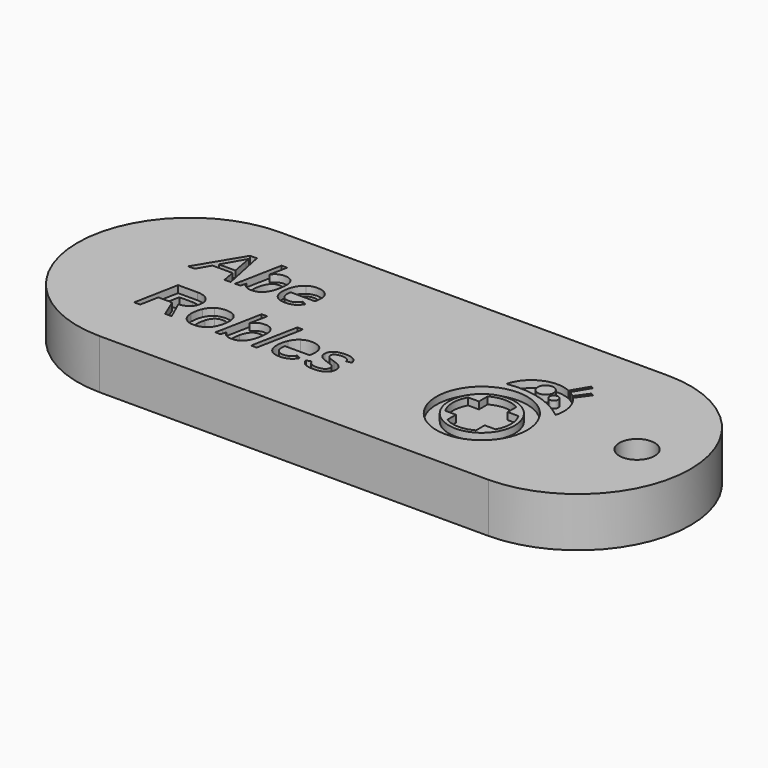
from build123d import *

# Parameters (mm, degrees)
F0_R         = 8.1541463089
F0_R_2       = 3.175
F1_DEPTH     = 8.89
F0_TEXT_SIZE = 11.5409836066
F2_DEPTH     = 7.62
F0_R_3       = 5.9091517201
F0_R_4       = 0.7843933306
F0_R_5       = 1.4228643603
F3_DEPTH     = 7.62
F4_DEPTH     = 8.89


# Not quite as in the source:
# - Text() gives the source's letters only with a copy of the font that has no kerning and outlines rounded to 1/6400 em; it was checked with that copy


with BuildPart() as f1:
    # F0 (on Top) → F1 (new body)
    with BuildSketch(Plane.XY):
        with BuildLine():
            ThreePointArc((34.925, -20.2309455037), (55.0719912037, 0), (34.925, 20.2309455037))
            Line((34.925, 20.2309455037), (34.7567415551, 20.2309455037))
            Line((34.7567415551, 20.2309455037), (-34.7567415551, 20.2309455037))
            Line((-34.7567415551, 20.2309455037), (-34.925, 20.2309455037))
            ThreePointArc((-34.925, 20.2309455037), (-55.0719912037, 0), (-34.925, -20.2309455037))
            Line((-34.925, -20.2309455037), (-34.7567415551, -20.2309455037))
            Line((-34.7567415551, -20.2309455037), (34.7567415551, -20.2309455037))
            Line((34.7567415551, -20.2309455037), (34.925, -20.2309455037))
        make_face()
        with BuildLine():
            Line((-30.8085259014, -9.1939333774), (-31.9698373768, -9.1939333774))
            Line((-31.9698373768, -9.1939333774), (-33.3385259014, -5.8975399348))
            Line((-33.3385259014, -5.8975399348), (-35.8234439342, -5.8975399348))
            Line((-35.8234439342, -5.8975399348), (-36.4600013112, -9.1939333774))
            Line((-36.4600013112, -9.1939333774), (-37.5365586883, -9.1939333774))
            Line((-37.5365586883, -9.1939333774), (-35.9983619669, -1.2540973119))
            Line((-35.9983619669, -1.2540973119), (-32.5486898358, -1.2540973119))
            add(Edge.make_bspline(
                [(-32.5486898358, -1.2540973119), (-31.3440996719, -1.2540973119), (-30.6281980325, -1.8284415742)],
                knots=[0, 0, 0, 1, 1, 1], degree=2))
            add(Edge.make_bspline(
                [(-30.6281980325, -1.8284415742), (-29.9122963932, -2.4027858364), (-29.9122963932, -3.3386874758)],
                knots=[0, 0, 0, 1, 1, 1], degree=2))
            add(Edge.make_bspline(
                [(-29.9122963932, -3.3386874758), (-29.9122963932, -4.3990153446), (-30.5209029505, -5.0184415742)],
                knots=[0, 0, 0, 1, 1, 1], degree=2))
            add(Edge.make_bspline(
                [(-30.5209029505, -5.0184415742), (-31.1295095079, -5.6378678037), (-32.3178701637, -5.8019661643)],
                knots=[0, 0, 0, 1, 1, 1], degree=2))
            Line((-32.3178701637, -5.8019661643), (-30.8085259014, -9.1939333774))
        make_face(mode=Mode.SUBTRACT)
        with BuildLine():
            add(Edge.make_bspline(
                [(-24.1300832784, -3.606474361), (-23.5052472128, -4.2240973119), (-23.5052472128, -5.3457366561)],
                knots=[0, 0, 0, 1, 1, 1], degree=2))
            add(Edge.make_bspline(
                [(-23.5052472128, -5.3457366561), (-23.5052472128, -6.0778678037), (-23.7306570489, -6.8695071479)],
                knots=[0, 0, 0, 1, 1, 1], degree=2))
            add(Edge.make_bspline(
                [(-23.7306570489, -6.8695071479), (-23.956066885, -7.6611464922), (-24.3753291801, -8.2102448528)],
                knots=[0, 0, 0, 1, 1, 1], degree=2))
            add(Edge.make_bspline(
                [(-24.3753291801, -8.2102448528), (-24.7945914751, -8.7593432135), (-25.4031980325, -9.0334415742)],
                knots=[0, 0, 0, 1, 1, 1], degree=2))
            add(Edge.make_bspline(
                [(-25.4031980325, -9.0334415742), (-26.0118045899, -9.3075399348), (-26.7908209833, -9.3075399348)],
                knots=[0, 0, 0, 1, 1, 1], degree=2))
            add(Edge.make_bspline(
                [(-26.7908209833, -9.3075399348), (-27.8944275407, -9.3075399348), (-28.5372963932, -8.6421300987)],
                knots=[0, 0, 0, 1, 1, 1], degree=2))
            add(Edge.make_bspline(
                [(-28.5372963932, -8.6421300987), (-29.1801652456, -7.9767202627), (-29.1801652456, -6.8334415742)],
                knots=[0, 0, 0, 1, 1, 1], degree=2))
            add(Edge.make_bspline(
                [(-29.1801652456, -6.8334415742), (-29.1567226227, -5.6829497709), (-28.7627062292, -4.7930317381)],
                knots=[0, 0, 0, 1, 1, 1], degree=2))
            add(Edge.make_bspline(
                [(-28.7627062292, -4.7930317381), (-28.3686898358, -3.9031137053), (-27.669919344, -3.4459825578)],
                knots=[0, 0, 0, 1, 1, 1], degree=2))
            add(Edge.make_bspline(
                [(-27.669919344, -3.4459825578), (-26.9711488522, -2.9888514102), (-25.9396734423, -2.9888514102)],
                knots=[0, 0, 0, 1, 1, 1], degree=2))
            add(Edge.make_bspline(
                [(-25.9396734423, -2.9888514102), (-24.754919344, -2.9888514102), (-24.1300832784, -3.606474361)],
                knots=[0, 0, 0, 1, 1, 1], degree=2))
        make_face(mode=Mode.SUBTRACT)
        with BuildLine():
            add(Edge.make_bspline(
                [(-20.0736078686, -3.2259825578), (-19.6173783604, -2.9834415742), (-18.9465586883, -2.9834415742)],
                knots=[0, 0, 0, 1, 1, 1], degree=2))
            add(Edge.make_bspline(
                [(-18.9465586883, -2.9834415742), (-18.0611488522, -2.9834415742), (-17.5679521309, -3.5163104266)],
                knots=[0, 0, 0, 1, 1, 1], degree=2))
            add(Edge.make_bspline(
                [(-17.5679521309, -3.5163104266), (-17.0747554096, -4.0491792791), (-17.0747554096, -4.9778678037)],
                knots=[0, 0, 0, 1, 1, 1], degree=2))
            add(Edge.make_bspline(
                [(-17.0747554096, -4.9778678037), (-17.0747554096, -6.1229497709), (-17.4218865571, -7.1959005905)],
                knots=[0, 0, 0, 1, 1, 1], degree=2))
            add(Edge.make_bspline(
                [(-17.4218865571, -7.1959005905), (-17.7690177046, -8.2688514102), (-18.3974603276, -8.7881956725)],
                knots=[0, 0, 0, 1, 1, 1], degree=2))
            add(Edge.make_bspline(
                [(-18.3974603276, -8.7881956725), (-19.0259029505, -9.3075399348), (-19.9996734423, -9.3075399348)],
                knots=[0, 0, 0, 1, 1, 1], degree=2))
            add(Edge.make_bspline(
                [(-19.9996734423, -9.3075399348), (-20.6939357374, -9.3075399348), (-21.127624262, -9.0136055086)],
                knots=[0, 0, 0, 1, 1, 1], degree=2))
            add(Edge.make_bspline(
                [(-21.127624262, -9.0136055086), (-21.5613127866, -8.7196710824), (-21.7416406555, -8.1913104266)],
                knots=[0, 0, 0, 1, 1, 1], degree=2))
            Line((-21.7416406555, -8.1913104266), (-21.7578701637, -8.1913104266))
            add(Edge.make_bspline(
                [(-21.7578701637, -8.1913104266), (-21.7975422948, -8.3986874758), (-21.8931160653, -8.7881956725)],
                knots=[0, 0, 0, 1, 1, 1], degree=2))
            add(Edge.make_bspline(
                [(-21.8931160653, -8.7881956725), (-21.9886898358, -9.1777038692), (-22.0013127866, -9.1939333774)],
                knots=[0, 0, 0, 1, 1, 1], degree=2))
            Line((-22.0013127866, -9.1939333774), (-22.9750832784, -9.1939333774))
            add(Edge.make_bspline(
                [(-22.9750832784, -9.1939333774), (-22.9480340981, -9.1091792791), (-22.8659849178, -8.7313923938)],
                knots=[0, 0, 0, 1, 1, 1], degree=2))
            add(Edge.make_bspline(
                [(-22.8659849178, -8.7313923938), (-22.7839357374, -8.3536055086), (-22.6991816391, -7.9370481315)],
                knots=[0, 0, 0, 1, 1, 1], degree=2))
            Line((-22.6991816391, -7.9370481315), (-21.3196734423, -0.8303268201))
            Line((-21.3196734423, -0.8303268201), (-20.3044275407, -0.8303268201))
            Line((-20.3044275407, -0.8303268201), (-20.771476721, -3.2142612463))
            add(Edge.make_bspline(
                [(-20.771476721, -3.2142612463), (-20.8165586883, -3.4739333774), (-20.9644275407, -4.0040973119)],
                knots=[0, 0, 0, 1, 1, 1], degree=2))
            Line((-20.9644275407, -4.0040973119), (-20.9409849178, -4.0040973119))
            add(Edge.make_bspline(
                [(-20.9409849178, -4.0040973119), (-20.5298373768, -3.4685235414), (-20.0736078686, -3.2259825578)],
                knots=[0, 0, 0, 1, 1, 1], degree=2))
        make_face(mode=Mode.SUBTRACT)
        with BuildLine():
            Line((-8.3018045899, -6.3591792791), (-12.7144275407, -6.3591792791))
            add(Edge.make_bspline(
                [(-12.7144275407, -6.3591792791), (-12.7486898358, -6.5557366561), (-12.764919344, -6.9957366561)],
                knots=[0, 0, 0, 1, 1, 1], degree=2))
            add(Edge.make_bspline(
                [(-12.764919344, -6.9957366561), (-12.764919344, -7.7459005905), (-12.3898373768, -8.1462284594)],
                knots=[0, 0, 0, 1, 1, 1], degree=2))
            add(Edge.make_bspline(
                [(-12.3898373768, -8.1462284594), (-12.0147554096, -8.5465563283), (-11.2609849178, -8.5465563283)],
                knots=[0, 0, 0, 1, 1, 1], degree=2))
            add(Edge.make_bspline(
                [(-11.2609849178, -8.5465563283), (-10.7145914751, -8.5465563283), (-10.2691816391, -8.276064525)],
                knots=[0, 0, 0, 1, 1, 1], degree=2))
            add(Edge.make_bspline(
                [(-10.2691816391, -8.276064525), (-9.823771803, -8.0055727217), (-9.574919344, -7.5367202627)],
                knots=[0, 0, 0, 1, 1, 1], degree=2))
            Line((-9.574919344, -7.5367202627), (-8.7977062292, -7.8919661643))
            add(Edge.make_bspline(
                [(-8.7977062292, -7.8919661643), (-9.2088537702, -8.6295071479), (-9.8427062292, -8.9685235414)],
                knots=[0, 0, 0, 1, 1, 1], degree=2))
            add(Edge.make_bspline(
                [(-9.8427062292, -8.9685235414), (-10.4765586883, -9.3075399348), (-11.3781980325, -9.3075399348)],
                knots=[0, 0, 0, 1, 1, 1], degree=2))
            add(Edge.make_bspline(
                [(-11.3781980325, -9.3075399348), (-12.5106570489, -9.3075399348), (-13.1390996719, -8.6790973119)],
                knots=[0, 0, 0, 1, 1, 1], degree=2))
            add(Edge.make_bspline(
                [(-13.1390996719, -8.6790973119), (-13.7675422948, -8.0506546889), (-13.7675422948, -6.9109825578)],
                knots=[0, 0, 0, 1, 1, 1], degree=2))
            add(Edge.make_bspline(
                [(-13.7675422948, -6.9109825578), (-13.7675422948, -5.7785235414), (-13.3681160653, -4.8795891151)],
                knots=[0, 0, 0, 1, 1, 1], degree=2))
            add(Edge.make_bspline(
                [(-13.3681160653, -4.8795891151), (-12.9686898358, -3.9806546889), (-12.241066885, -3.4820481315)],
                knots=[0, 0, 0, 1, 1, 1], degree=2))
            add(Edge.make_bspline(
                [(-12.241066885, -3.4820481315), (-11.5134439342, -2.9834415742), (-10.6063947538, -2.9834415742)],
                knots=[0, 0, 0, 1, 1, 1], degree=2))
            add(Edge.make_bspline(
                [(-10.6063947538, -2.9834415742), (-9.4522963932, -2.9834415742), (-8.8094275407, -3.5640973119)],
                knots=[0, 0, 0, 1, 1, 1], degree=2))
            add(Edge.make_bspline(
                [(-8.8094275407, -3.5640973119), (-8.1665586883, -4.1447530496), (-8.1665586883, -5.2032776397)],
                knots=[0, 0, 0, 1, 1, 1], degree=2))
            add(Edge.make_bspline(
                [(-8.1665586883, -5.2032776397), (-8.1665586883, -5.7965563283), (-8.3018045899, -6.3591792791)],
                knots=[0, 0, 0, 1, 1, 1], degree=2))
        make_face(mode=Mode.SUBTRACT)
        with BuildLine():
            add(Edge.make_bspline(
                [(-2.8315586883, -6.6639333774), (-2.6286898358, -6.9795071479), (-2.6286898358, -7.4068841971)],
                knots=[0, 0, 0, 1, 1, 1], degree=2))
            add(Edge.make_bspline(
                [(-2.6286898358, -7.4068841971), (-2.6286898358, -8.3211464922), (-3.3274603276, -8.8143432135)],
                knots=[0, 0, 0, 1, 1, 1], degree=2))
            add(Edge.make_bspline(
                [(-3.3274603276, -8.8143432135), (-4.0262308194, -9.3075399348), (-5.3444275407, -9.3075399348)],
                knots=[0, 0, 0, 1, 1, 1], degree=2))
            add(Edge.make_bspline(
                [(-5.3444275407, -9.3075399348), (-6.3254111473, -9.3075399348), (-6.9024603276, -8.9775399348)],
                knots=[0, 0, 0, 1, 1, 1], degree=2))
            add(Edge.make_bspline(
                [(-6.9024603276, -8.9775399348), (-7.4795095079, -8.6475399348), (-7.7103291801, -7.9370481315)],
                knots=[0, 0, 0, 1, 1, 1], degree=2))
            Line((-7.7103291801, -7.9370481315), (-6.882624262, -7.621474361))
            add(Edge.make_bspline(
                [(-6.882624262, -7.621474361), (-6.6968865571, -8.1173760004), (-6.3046734423, -8.3427858364)],
                knots=[0, 0, 0, 1, 1, 1], degree=2))
            add(Edge.make_bspline(
                [(-6.3046734423, -8.3427858364), (-5.9124603276, -8.5681956725), (-5.2542636063, -8.5681956725)],
                knots=[0, 0, 0, 1, 1, 1], degree=2))
            add(Edge.make_bspline(
                [(-5.2542636063, -8.5681956725), (-4.4481980325, -8.5681956725), (-4.0307390161, -8.2949989512)],
                knots=[0, 0, 0, 1, 1, 1], degree=2))
            add(Edge.make_bspline(
                [(-4.0307390161, -8.2949989512), (-3.6132799997, -8.0218022299), (-3.6132799997, -7.4970481315)],
                knots=[0, 0, 0, 1, 1, 1], degree=2))
            add(Edge.make_bspline(
                [(-3.6132799997, -7.4970481315), (-3.6132799997, -7.1490153446), (-3.9009029505, -6.9145891151)],
                knots=[0, 0, 0, 1, 1, 1], degree=2))
            add(Edge.make_bspline(
                [(-3.9009029505, -6.9145891151), (-4.1885259014, -6.6801628856), (-5.1190177046, -6.3934415742)],
                knots=[0, 0, 0, 1, 1, 1], degree=2))
            add(Edge.make_bspline(
                [(-5.1190177046, -6.3934415742), (-5.8403291801, -6.157212066), (-6.2009849178, -5.9318022299)],
                knots=[0, 0, 0, 1, 1, 1], degree=2))
            add(Edge.make_bspline(
                [(-6.2009849178, -5.9318022299), (-6.5616406555, -5.7063923938), (-6.7527881964, -5.4043432135)],
                knots=[0, 0, 0, 1, 1, 1], degree=2))
            add(Edge.make_bspline(
                [(-6.7527881964, -5.4043432135), (-6.9439357374, -5.1022940332), (-6.9439357374, -4.7019661643)],
                knots=[0, 0, 0, 1, 1, 1], degree=2))
            add(Edge.make_bspline(
                [(-6.9439357374, -4.7019661643), (-6.9439357374, -3.8850809184), (-6.2902472128, -3.4432776397)],
                knots=[0, 0, 0, 1, 1, 1], degree=2))
            add(Edge.make_bspline(
                [(-6.2902472128, -3.4432776397), (-5.6365586883, -3.001474361), (-4.4481980325, -3.001474361)],
                knots=[0, 0, 0, 1, 1, 1], degree=2))
            add(Edge.make_bspline(
                [(-4.4481980325, -3.001474361), (-2.453771803, -3.001474361), (-2.204919344, -4.4368841971)],
                knots=[0, 0, 0, 1, 1, 1], degree=2))
            Line((-2.204919344, -4.4368841971), (-3.1245914751, -4.5793432135))
            add(Edge.make_bspline(
                [(-3.1245914751, -4.5793432135), (-3.247214426, -4.1339333774), (-3.5916406555, -3.936474361)],
                knots=[0, 0, 0, 1, 1, 1], degree=2))
            add(Edge.make_bspline(
                [(-3.5916406555, -3.936474361), (-3.936066885, -3.7390153446), (-4.514919344, -3.7390153446)],
                knots=[0, 0, 0, 1, 1, 1], degree=2))
            add(Edge.make_bspline(
                [(-4.514919344, -3.7390153446), (-5.2145914751, -3.7390153446), (-5.5896734423, -3.9617202627)],
                knots=[0, 0, 0, 1, 1, 1], degree=2))
            add(Edge.make_bspline(
                [(-5.5896734423, -3.9617202627), (-5.9647554096, -4.1844251807), (-5.9647554096, -4.5901628856)],
                knots=[0, 0, 0, 1, 1, 1], degree=2))
            add(Edge.make_bspline(
                [(-5.9647554096, -4.5901628856), (-5.9647554096, -4.8263923938), (-5.8457390161, -4.9895891151)],
                knots=[0, 0, 0, 1, 1, 1], degree=2))
            add(Edge.make_bspline(
                [(-5.8457390161, -4.9895891151), (-5.7267226227, -5.1527858364), (-5.5040177046, -5.279916984)],
                knots=[0, 0, 0, 1, 1, 1], degree=2))
            add(Edge.make_bspline(
                [(-5.5040177046, -5.279916984), (-5.2813127866, -5.4070481315), (-4.4770504915, -5.6613104266)],
                knots=[0, 0, 0, 1, 1, 1], degree=2))
            add(Edge.make_bspline(
                [(-4.4770504915, -5.6613104266), (-3.7611488522, -5.8867202627), (-3.3977881964, -6.1175399348)],
                knots=[0, 0, 0, 1, 1, 1], degree=2))
            add(Edge.make_bspline(
                [(-3.3977881964, -6.1175399348), (-3.0344275407, -6.3483596069), (-2.8315586883, -6.6639333774)],
                knots=[0, 0, 0, 1, 1, 1], degree=2))
        make_face(mode=Mode.SUBTRACT)
        Polygon((-15.5257390161, -9.1939333774), (-16.5355750817, -9.1939333774), (-14.912624262, -0.8303268201), (-13.8973783604, -0.8303268201), align=None, mode=Mode.SUBTRACT)
        with Locations((21.6285008937, -5.0627232608)):
            Circle(F0_R, mode=Mode.SUBTRACT)
        with Locations((45.4701632261, 0)):
            Circle(F0_R_2, mode=Mode.SUBTRACT)
        Polygon((-30.8139357374, 4.0781977701), (-31.9121324587, 4.0781977701), (-32.3359029505, 6.4008207209), (-35.9370504915, 6.4008207209), (-37.2895095079, 4.0781977701), (-38.4616406555, 4.0781977701), (-33.6829521309, 12.0180338357), (-32.4585259014, 12.0180338357), align=None, mode=Mode.SUBTRACT)
        with BuildLine():
            Line((-17.9204931145, 6.9129518685), (-22.3331160653, 6.9129518685))
            add(Edge.make_bspline(
                [(-22.3331160653, 6.9129518685), (-22.3673783604, 6.7163944914), (-22.3836078686, 6.2763944914)],
                knots=[0, 0, 0, 1, 1, 1], degree=2))
            add(Edge.make_bspline(
                [(-22.3836078686, 6.2763944914), (-22.3836078686, 5.526230557), (-22.0085259014, 5.1259026881)],
                knots=[0, 0, 0, 1, 1, 1], degree=2))
            add(Edge.make_bspline(
                [(-22.0085259014, 5.1259026881), (-21.6334439342, 4.7255748193), (-20.8796734423, 4.7255748193)],
                knots=[0, 0, 0, 1, 1, 1], degree=2))
            add(Edge.make_bspline(
                [(-20.8796734423, 4.7255748193), (-20.3332799997, 4.7255748193), (-19.8878701637, 4.9960666226)],
                knots=[0, 0, 0, 1, 1, 1], degree=2))
            add(Edge.make_bspline(
                [(-19.8878701637, 4.9960666226), (-19.4424603276, 5.2665584258), (-19.1936078686, 5.7354108849)],
                knots=[0, 0, 0, 1, 1, 1], degree=2))
            Line((-19.1936078686, 5.7354108849), (-18.4163947538, 5.3801649832))
            add(Edge.make_bspline(
                [(-18.4163947538, 5.3801649832), (-18.8275422948, 4.6426239996), (-19.4613947538, 4.3036076062)],
                knots=[0, 0, 0, 1, 1, 1], degree=2))
            add(Edge.make_bspline(
                [(-19.4613947538, 4.3036076062), (-20.0952472128, 3.9645912127), (-20.9968865571, 3.9645912127)],
                knots=[0, 0, 0, 1, 1, 1], degree=2))
            add(Edge.make_bspline(
                [(-20.9968865571, 3.9645912127), (-22.1293455735, 3.9645912127), (-22.7577881964, 4.5930338357)],
                knots=[0, 0, 0, 1, 1, 1], degree=2))
            add(Edge.make_bspline(
                [(-22.7577881964, 4.5930338357), (-23.3862308194, 5.2214764586), (-23.3862308194, 6.3611485898)],
                knots=[0, 0, 0, 1, 1, 1], degree=2))
            add(Edge.make_bspline(
                [(-23.3862308194, 6.3611485898), (-23.3862308194, 7.4936076062), (-22.9868045899, 8.3925420324)],
                knots=[0, 0, 0, 1, 1, 1], degree=2))
            add(Edge.make_bspline(
                [(-22.9868045899, 8.3925420324), (-22.5873783604, 9.2914764586), (-21.8597554096, 9.790083016)],
                knots=[0, 0, 0, 1, 1, 1], degree=2))
            add(Edge.make_bspline(
                [(-21.8597554096, 9.790083016), (-21.1321324587, 10.2886895734), (-20.2250832784, 10.2886895734)],
                knots=[0, 0, 0, 1, 1, 1], degree=2))
            add(Edge.make_bspline(
                [(-20.2250832784, 10.2886895734), (-19.0709849178, 10.2886895734), (-18.4281160653, 9.7080338357)],
                knots=[0, 0, 0, 1, 1, 1], degree=2))
            add(Edge.make_bspline(
                [(-18.4281160653, 9.7080338357), (-17.7852472128, 9.127378098), (-17.7852472128, 8.0688535078)],
                knots=[0, 0, 0, 1, 1, 1], degree=2))
            add(Edge.make_bspline(
                [(-17.7852472128, 8.0688535078), (-17.7852472128, 7.4755748193), (-17.9204931145, 6.9129518685)],
                knots=[0, 0, 0, 1, 1, 1], degree=2))
        make_face(mode=Mode.SUBTRACT)
        with BuildLine():
            add(Edge.make_bspline(
                [(-27.1280340981, 10.0461485898), (-26.6718045899, 10.2886895734), (-26.0009849178, 10.2886895734)],
                knots=[0, 0, 0, 1, 1, 1], degree=2))
            add(Edge.make_bspline(
                [(-26.0009849178, 10.2886895734), (-25.1155750817, 10.2886895734), (-24.6223783604, 9.7558207209)],
                knots=[0, 0, 0, 1, 1, 1], degree=2))
            add(Edge.make_bspline(
                [(-24.6223783604, 9.7558207209), (-24.1291816391, 9.2229518685), (-24.1291816391, 8.2942633439)],
                knots=[0, 0, 0, 1, 1, 1], degree=2))
            add(Edge.make_bspline(
                [(-24.1291816391, 8.2942633439), (-24.1291816391, 7.1491813767), (-24.4763127866, 6.076230557)],
                knots=[0, 0, 0, 1, 1, 1], degree=2))
            add(Edge.make_bspline(
                [(-24.4763127866, 6.076230557), (-24.8234439342, 5.0032797373), (-25.4518865571, 4.483935475)],
                knots=[0, 0, 0, 1, 1, 1], degree=2))
            add(Edge.make_bspline(
                [(-25.4518865571, 4.483935475), (-26.0803291801, 3.9645912127), (-27.0540996719, 3.9645912127)],
                knots=[0, 0, 0, 1, 1, 1], degree=2))
            add(Edge.make_bspline(
                [(-27.0540996719, 3.9645912127), (-27.7483619669, 3.9645912127), (-28.1820504915, 4.258525639)],
                knots=[0, 0, 0, 1, 1, 1], degree=2))
            add(Edge.make_bspline(
                [(-28.1820504915, 4.258525639), (-28.6157390161, 4.5524600652), (-28.796066885, 5.0808207209)],
                knots=[0, 0, 0, 1, 1, 1], degree=2))
            Line((-28.796066885, 5.0808207209), (-28.8122963932, 5.0808207209))
            add(Edge.make_bspline(
                [(-28.8122963932, 5.0808207209), (-28.8519685243, 4.8734436717), (-28.9475422948, 4.483935475)],
                knots=[0, 0, 0, 1, 1, 1], degree=2))
            add(Edge.make_bspline(
                [(-28.9475422948, 4.483935475), (-29.0431160653, 4.0944272783), (-29.0557390161, 4.0781977701)],
                knots=[0, 0, 0, 1, 1, 1], degree=2))
            Line((-29.0557390161, 4.0781977701), (-30.0295095079, 4.0781977701))
            add(Edge.make_bspline(
                [(-30.0295095079, 4.0781977701), (-30.0024603276, 4.1629518685), (-29.9204111473, 4.5407387537)],
                knots=[0, 0, 0, 1, 1, 1], degree=2))
            add(Edge.make_bspline(
                [(-29.9204111473, 4.5407387537), (-29.8383619669, 4.918525639), (-29.7536078686, 5.335083016)],
                knots=[0, 0, 0, 1, 1, 1], degree=2))
            Line((-29.7536078686, 5.335083016), (-28.3740996719, 12.4418043275))
            Line((-28.3740996719, 12.4418043275), (-27.3588537702, 12.4418043275))
            Line((-27.3588537702, 12.4418043275), (-27.8259029505, 10.0578699013))
            add(Edge.make_bspline(
                [(-27.8259029505, 10.0578699013), (-27.8709849178, 9.7981977701), (-28.0188537702, 9.2680338357)],
                knots=[0, 0, 0, 1, 1, 1], degree=2))
            Line((-28.0188537702, 9.2680338357), (-27.9954111473, 9.2680338357))
            add(Edge.make_bspline(
                [(-27.9954111473, 9.2680338357), (-27.5842636063, 9.8036076062), (-27.1280340981, 10.0461485898)],
                knots=[0, 0, 0, 1, 1, 1], degree=2))
        make_face(mode=Mode.SUBTRACT)
        with BuildLine():
            ThreePointArc((28.6599894676, 6.6070121564), (30.0717011738, 3.9846779943), (30.0103016113, 1.0071292554))
            ThreePointArc((30.0103016113, 1.0071292554), (24.6999169301, 3.7792163681), (18.7175344568, 4.0886551586))
            ThreePointArc((18.7175344568, 4.0886551586), (21.8588782947, 7.8942806377), (26.7932641168, 7.9458844505))
            Line((26.7932641168, 7.9458844505), (28.5554677248, 10.9033929184))
            Line((28.5554677248, 10.9033929184), (29.0221851319, 10.6823155656))
            Line((29.0221851319, 10.6823155656), (27.253003791, 7.71309636))
            ThreePointArc((27.253003791, 7.71309636), (27.7734789762, 7.3828360458), (28.256335807, 6.9996708405))
            Line((28.256335807, 6.9996708405), (29.8575228984, 9.2063825416))
            Line((29.8575228984, 9.2063825416), (30.3699612103, 8.9636478509))
            Line((30.3699612103, 8.9636478509), (28.6599894676, 6.6070121564))
        make_face(mode=Mode.SUBTRACT)
    extrude(amount=F1_DEPTH)

    # F0 (on Top) → F3 (join)
    with BuildSketch(Plane.XY):
        with Locations((21.6285008937, -5.0627232608)):
            Circle(F0_R)
        with Locations((21.6285008937, -5.0627232608)):
            Circle(F0_R_3, mode=Mode.SUBTRACT)
        with BuildLine():
            ThreePointArc((18.7175344568, 4.0886551586), (24.6999169301, 3.7792163681), (30.0103016113, 1.0071292554))
            ThreePointArc((30.0103016113, 1.0071292554), (30.0717011738, 3.9846779943), (28.6599894676, 6.6070121564))
            Line((28.6599894676, 6.6070121564), (30.3699612103, 8.9636478509))
            Line((30.3699612103, 8.9636478509), (29.8575228984, 9.2063825416))
            Line((29.8575228984, 9.2063825416), (28.256335807, 6.9996708405))
            ThreePointArc((28.256335807, 6.9996708405), (27.7734789762, 7.3828360458), (27.253003791, 7.71309636))
            Line((27.253003791, 7.71309636), (29.0221851319, 10.6823155656))
            Line((29.0221851319, 10.6823155656), (28.5554677248, 10.9033929184))
            Line((28.5554677248, 10.9033929184), (26.7932641168, 7.9458844505))
            ThreePointArc((26.7932641168, 7.9458844505), (21.8588782947, 7.8942806377), (18.7175344568, 4.0886551586))
        make_face()
        with Locations((26.6166795045, 4.8779863864)):
            Circle(F0_R_4, mode=Mode.SUBTRACT)
        with Locations((24.1906922311, 6.0710948892)):
            Circle(F0_R_5, mode=Mode.SUBTRACT)
    extrude(amount=F3_DEPTH)


with BuildPart() as f1b:
    # F0 (on Top) → F1, piece 2 (new body)
    with BuildSketch(Plane.XY):
        with BuildLine():
            Line((-33.0680340981, 10.3554108849), (-33.2140996719, 11.2065584258))
            add(Edge.make_bspline(
                [(-33.2140996719, 11.2065584258), (-33.2880340981, 11.0604928521), (-33.4232799997, 10.8179518685)],
                knots=[0, 0, 0, 1, 1, 1], degree=2))
            add(Edge.make_bspline(
                [(-33.4232799997, 10.8179518685), (-33.5585259014, 10.5754108849), (-35.4627881964, 7.2393453111)],
                knots=[0, 0, 0, 1, 1, 1], degree=2))
            Line((-35.4627881964, 7.2393453111), (-32.4927881964, 7.2393453111))
            Line((-32.4927881964, 7.2393453111), (-33.0680340981, 10.3554108849))
        make_face()
    extrude(amount=F1_DEPTH)


with BuildPart() as f2:
    # F0 (on Top) → F2 (new body)
    with BuildSketch(Plane.XY):
        with Locations((-37.8918045899, 4.0781977701)):
            Text('Abe', F0_TEXT_SIZE, font='Arimo', font_style=FontStyle.ITALIC, text_align=(TextAlign.LEFT, TextAlign.BOTTOM))
        with BuildLine():
            Line((-33.3385259014, -5.8975399348), (-31.9698373768, -9.1939333774))
            Line((-31.9698373768, -9.1939333774), (-30.8085259014, -9.1939333774))
            Line((-30.8085259014, -9.1939333774), (-32.3178701637, -5.8019661643))
            add(Edge.make_bspline(
                [(-30.5209029505, -5.0184415742), (-31.1295095079, -5.6378678037), (-32.3178701637, -5.8019661643)],
                knots=[0, 0, 0, 1, 1, 1], degree=2))
            add(Edge.make_bspline(
                [(-29.9122963932, -3.3386874758), (-29.9122963932, -4.3990153446), (-30.5209029505, -5.0184415742)],
                knots=[0, 0, 0, 1, 1, 1], degree=2))
            add(Edge.make_bspline(
                [(-30.6281980325, -1.8284415742), (-29.9122963932, -2.4027858364), (-29.9122963932, -3.3386874758)],
                knots=[0, 0, 0, 1, 1, 1], degree=2))
            add(Edge.make_bspline(
                [(-32.5486898358, -1.2540973119), (-31.3440996719, -1.2540973119), (-30.6281980325, -1.8284415742)],
                knots=[0, 0, 0, 1, 1, 1], degree=2))
            Line((-32.5486898358, -1.2540973119), (-35.9983619669, -1.2540973119))
            Line((-35.9983619669, -1.2540973119), (-37.5365586883, -9.1939333774))
            Line((-37.5365586883, -9.1939333774), (-36.4600013112, -9.1939333774))
            Line((-36.4600013112, -9.1939333774), (-35.8234439342, -5.8975399348))
            Line((-35.8234439342, -5.8975399348), (-33.3385259014, -5.8975399348))
        make_face()
        with BuildLine():
            add(Edge.make_bspline(
                [(-33.062624262, -5.0463923938), (-32.0419685243, -5.0463923938), (-31.5235259014, -4.6208186233)],
                knots=[0, 0, 0, 1, 1, 1], degree=2))
            Line((-33.062624262, -5.0463923938), (-35.6539357374, -5.0463923938))
            Line((-35.6539357374, -5.0463923938), (-35.0859029505, -2.116064525))
            Line((-35.0859029505, -2.116064525), (-32.6785259014, -2.116064525))
            add(Edge.make_bspline(
                [(-31.4252472128, -2.4541792791), (-31.8454111473, -2.116064525), (-32.6785259014, -2.116064525)],
                knots=[0, 0, 0, 1, 1, 1], degree=2))
            add(Edge.make_bspline(
                [(-31.0050832784, -3.4234415742), (-31.0050832784, -2.7922940332), (-31.4252472128, -2.4541792791)],
                knots=[0, 0, 0, 1, 1, 1], degree=2))
            add(Edge.make_bspline(
                [(-31.5235259014, -4.6208186233), (-31.0050832784, -4.1952448528), (-31.0050832784, -3.4234415742)],
                knots=[0, 0, 0, 1, 1, 1], degree=2))
        make_face(mode=Mode.SUBTRACT)
        with BuildLine():
            add(Edge.make_bspline(
                [(-23.5052472128, -5.3457366561), (-23.5052472128, -6.0778678037), (-23.7306570489, -6.8695071479)],
                knots=[0, 0, 0, 1, 1, 1], degree=2))
            add(Edge.make_bspline(
                [(-24.1300832784, -3.606474361), (-23.5052472128, -4.2240973119), (-23.5052472128, -5.3457366561)],
                knots=[0, 0, 0, 1, 1, 1], degree=2))
            add(Edge.make_bspline(
                [(-25.9396734423, -2.9888514102), (-24.754919344, -2.9888514102), (-24.1300832784, -3.606474361)],
                knots=[0, 0, 0, 1, 1, 1], degree=2))
            add(Edge.make_bspline(
                [(-27.669919344, -3.4459825578), (-26.9711488522, -2.9888514102), (-25.9396734423, -2.9888514102)],
                knots=[0, 0, 0, 1, 1, 1], degree=2))
            add(Edge.make_bspline(
                [(-28.7627062292, -4.7930317381), (-28.3686898358, -3.9031137053), (-27.669919344, -3.4459825578)],
                knots=[0, 0, 0, 1, 1, 1], degree=2))
            add(Edge.make_bspline(
                [(-29.1801652456, -6.8334415742), (-29.1567226227, -5.6829497709), (-28.7627062292, -4.7930317381)],
                knots=[0, 0, 0, 1, 1, 1], degree=2))
            add(Edge.make_bspline(
                [(-28.5372963932, -8.6421300987), (-29.1801652456, -7.9767202627), (-29.1801652456, -6.8334415742)],
                knots=[0, 0, 0, 1, 1, 1], degree=2))
            add(Edge.make_bspline(
                [(-26.7908209833, -9.3075399348), (-27.8944275407, -9.3075399348), (-28.5372963932, -8.6421300987)],
                knots=[0, 0, 0, 1, 1, 1], degree=2))
            add(Edge.make_bspline(
                [(-25.4031980325, -9.0334415742), (-26.0118045899, -9.3075399348), (-26.7908209833, -9.3075399348)],
                knots=[0, 0, 0, 1, 1, 1], degree=2))
            add(Edge.make_bspline(
                [(-24.3753291801, -8.2102448528), (-24.7945914751, -8.7593432135), (-25.4031980325, -9.0334415742)],
                knots=[0, 0, 0, 1, 1, 1], degree=2))
            add(Edge.make_bspline(
                [(-23.7306570489, -6.8695071479), (-23.956066885, -7.6611464922), (-24.3753291801, -8.2102448528)],
                knots=[0, 0, 0, 1, 1, 1], degree=2))
        make_face()
        with BuildLine():
            add(Edge.make_bspline(
                [(-24.5529521309, -5.3457366561), (-24.5529521309, -3.7336055086), (-25.9504931145, -3.7336055086)],
                knots=[0, 0, 0, 1, 1, 1], degree=2))
            add(Edge.make_bspline(
                [(-24.7477062292, -6.6972940332), (-24.5818045899, -6.0544251807), (-24.5529521309, -5.3457366561)],
                knots=[0, 0, 0, 1, 1, 1], degree=2))
            add(Edge.make_bspline(
                [(-25.1786898358, -7.7540153446), (-24.9136078686, -7.3401628856), (-24.7477062292, -6.6972940332)],
                knots=[0, 0, 0, 1, 1, 1], degree=2))
            add(Edge.make_bspline(
                [(-25.7954111473, -8.362621902), (-25.443771803, -8.1678678037), (-25.1786898358, -7.7540153446)],
                knots=[0, 0, 0, 1, 1, 1], degree=2))
            add(Edge.make_bspline(
                [(-26.7277062292, -8.5573760004), (-26.1470504915, -8.5573760004), (-25.7954111473, -8.362621902)],
                knots=[0, 0, 0, 1, 1, 1], degree=2))
            add(Edge.make_bspline(
                [(-27.7754111473, -8.1200809184), (-27.4147554096, -8.5573760004), (-26.7277062292, -8.5573760004)],
                knots=[0, 0, 0, 1, 1, 1], degree=2))
            add(Edge.make_bspline(
                [(-28.136066885, -6.8496710824), (-28.136066885, -7.6827858364), (-27.7754111473, -8.1200809184)],
                knots=[0, 0, 0, 1, 1, 1], degree=2))
            add(Edge.make_bspline(
                [(-27.8827062292, -5.3105727217), (-28.136066885, -6.104916984), (-28.136066885, -6.8496710824)],
                knots=[0, 0, 0, 1, 1, 1], degree=2))
            add(Edge.make_bspline(
                [(-27.1704111473, -4.124916984), (-27.6293455735, -4.5162284594), (-27.8827062292, -5.3105727217)],
                knots=[0, 0, 0, 1, 1, 1], degree=2))
            add(Edge.make_bspline(
                [(-25.9504931145, -3.7336055086), (-26.711476721, -3.7336055086), (-27.1704111473, -4.124916984)],
                knots=[0, 0, 0, 1, 1, 1], degree=2))
        make_face(mode=Mode.SUBTRACT)
        with BuildLine():
            add(Edge.make_bspline(
                [(-18.9465586883, -2.9834415742), (-18.0611488522, -2.9834415742), (-17.5679521309, -3.5163104266)],
                knots=[0, 0, 0, 1, 1, 1], degree=2))
            add(Edge.make_bspline(
                [(-20.0736078686, -3.2259825578), (-19.6173783604, -2.9834415742), (-18.9465586883, -2.9834415742)],
                knots=[0, 0, 0, 1, 1, 1], degree=2))
            add(Edge.make_bspline(
                [(-20.9409849178, -4.0040973119), (-20.5298373768, -3.4685235414), (-20.0736078686, -3.2259825578)],
                knots=[0, 0, 0, 1, 1, 1], degree=2))
            Line((-20.9409849178, -4.0040973119), (-20.9644275407, -4.0040973119))
            add(Edge.make_bspline(
                [(-20.771476721, -3.2142612463), (-20.8165586883, -3.4739333774), (-20.9644275407, -4.0040973119)],
                knots=[0, 0, 0, 1, 1, 1], degree=2))
            Line((-20.771476721, -3.2142612463), (-20.3044275407, -0.8303268201))
            Line((-20.3044275407, -0.8303268201), (-21.3196734423, -0.8303268201))
            Line((-21.3196734423, -0.8303268201), (-22.6991816391, -7.9370481315))
            add(Edge.make_bspline(
                [(-22.8659849178, -8.7313923938), (-22.7839357374, -8.3536055086), (-22.6991816391, -7.9370481315)],
                knots=[0, 0, 0, 1, 1, 1], degree=2))
            add(Edge.make_bspline(
                [(-22.9750832784, -9.1939333774), (-22.9480340981, -9.1091792791), (-22.8659849178, -8.7313923938)],
                knots=[0, 0, 0, 1, 1, 1], degree=2))
            Line((-22.9750832784, -9.1939333774), (-22.0013127866, -9.1939333774))
            add(Edge.make_bspline(
                [(-21.8931160653, -8.7881956725), (-21.9886898358, -9.1777038692), (-22.0013127866, -9.1939333774)],
                knots=[0, 0, 0, 1, 1, 1], degree=2))
            add(Edge.make_bspline(
                [(-21.7578701637, -8.1913104266), (-21.7975422948, -8.3986874758), (-21.8931160653, -8.7881956725)],
                knots=[0, 0, 0, 1, 1, 1], degree=2))
            Line((-21.7578701637, -8.1913104266), (-21.7416406555, -8.1913104266))
            add(Edge.make_bspline(
                [(-21.127624262, -9.0136055086), (-21.5613127866, -8.7196710824), (-21.7416406555, -8.1913104266)],
                knots=[0, 0, 0, 1, 1, 1], degree=2))
            add(Edge.make_bspline(
                [(-19.9996734423, -9.3075399348), (-20.6939357374, -9.3075399348), (-21.127624262, -9.0136055086)],
                knots=[0, 0, 0, 1, 1, 1], degree=2))
            add(Edge.make_bspline(
                [(-18.3974603276, -8.7881956725), (-19.0259029505, -9.3075399348), (-19.9996734423, -9.3075399348)],
                knots=[0, 0, 0, 1, 1, 1], degree=2))
            add(Edge.make_bspline(
                [(-17.4218865571, -7.1959005905), (-17.7690177046, -8.2688514102), (-18.3974603276, -8.7881956725)],
                knots=[0, 0, 0, 1, 1, 1], degree=2))
            add(Edge.make_bspline(
                [(-17.0747554096, -4.9778678037), (-17.0747554096, -6.1229497709), (-17.4218865571, -7.1959005905)],
                knots=[0, 0, 0, 1, 1, 1], degree=2))
            add(Edge.make_bspline(
                [(-17.5679521309, -3.5163104266), (-17.0747554096, -4.0491792791), (-17.0747554096, -4.9778678037)],
                knots=[0, 0, 0, 1, 1, 1], degree=2))
        make_face()
        with BuildLine():
            add(Edge.make_bspline(
                [(-19.2386898358, -3.7678678037), (-19.7977062292, -3.7678678037), (-20.1944275407, -3.9959825578)],
                knots=[0, 0, 0, 1, 1, 1], degree=2))
            add(Edge.make_bspline(
                [(-18.4001652456, -4.1168022299), (-18.6652472128, -3.7678678037), (-19.2386898358, -3.7678678037)],
                knots=[0, 0, 0, 1, 1, 1], degree=2))
            add(Edge.make_bspline(
                [(-18.1350832784, -5.1590973119), (-18.1350832784, -4.4657366561), (-18.4001652456, -4.1168022299)],
                knots=[0, 0, 0, 1, 1, 1], degree=2))
            add(Edge.make_bspline(
                [(-18.3659029505, -6.7793432135), (-18.1350832784, -5.8524579676), (-18.1350832784, -5.1590973119)],
                knots=[0, 0, 0, 1, 1, 1], degree=2))
            add(Edge.make_bspline(
                [(-19.0024603276, -8.1318022299), (-18.5967226227, -7.7062284594), (-18.3659029505, -6.7793432135)],
                knots=[0, 0, 0, 1, 1, 1], degree=2))
            add(Edge.make_bspline(
                [(-20.1078701637, -8.5573760004), (-19.4081980325, -8.5573760004), (-19.0024603276, -8.1318022299)],
                knots=[0, 0, 0, 1, 1, 1], degree=2))
            add(Edge.make_bspline(
                [(-21.1023783604, -8.1651628856), (-20.7444275407, -8.5573760004), (-20.1078701637, -8.5573760004)],
                knots=[0, 0, 0, 1, 1, 1], degree=2))
            add(Edge.make_bspline(
                [(-21.4603291801, -7.0696710824), (-21.4603291801, -7.7729497709), (-21.1023783604, -8.1651628856)],
                knots=[0, 0, 0, 1, 1, 1], degree=2))
            add(Edge.make_bspline(
                [(-21.3025422948, -5.832621902), (-21.4603291801, -6.5232776397), (-21.4603291801, -7.0696710824)],
                knots=[0, 0, 0, 1, 1, 1], degree=2))
            add(Edge.make_bspline(
                [(-20.8679521309, -4.6830317381), (-21.1447554096, -5.1419661643), (-21.3025422948, -5.832621902)],
                knots=[0, 0, 0, 1, 1, 1], degree=2))
            add(Edge.make_bspline(
                [(-20.1944275407, -3.9959825578), (-20.5911488522, -4.2240973119), (-20.8679521309, -4.6830317381)],
                knots=[0, 0, 0, 1, 1, 1], degree=2))
        make_face(mode=Mode.SUBTRACT)
    extrude(amount=F2_DEPTH)


with BuildPart() as f3:
    # F0 (on Top) → F3, piece 2 (new body)
    with BuildSketch(Plane.XY):
        with BuildLine():
            Line((19.0458682724, -2.4800893608), (17.0969750505, -2.4800893608))
            ThreePointArc((17.0969750505, -2.4800893608), (16.4126860648, -5.0627232608), (17.0969750505, -7.6453571608))
            Line((17.0969750505, -7.6453571608), (19.0458682724, -7.6453571608))
            Line((19.0458682724, -7.6453571608), (19.0458682724, -9.5942498328))
            ThreePointArc((19.0458682724, -9.5942498328), (21.6285008937, -10.2785380897), (24.211133515, -9.5942498328))
            Line((24.211133515, -9.5942498328), (24.211133515, -7.6453571608))
            Line((24.211133515, -7.6453571608), (26.1600267369, -7.6453571608))
            ThreePointArc((26.1600267369, -7.6453571608), (26.8443157226, -5.0627232608), (26.1600267369, -2.4800893608))
            Line((26.1600267369, -2.4800893608), (24.211133515, -2.4800893608))
            Line((24.211133515, -2.4800893608), (24.211133515, -0.5311966889))
            ThreePointArc((24.211133515, -0.5311966889), (21.6285008937, 0.153091568), (19.0458682724, -0.5311966889))
            Line((19.0458682724, -0.5311966889), (19.0458682724, -2.4800893608))
        make_face()
    extrude(amount=F3_DEPTH)


with BuildPart() as f4:
    # F0 (on Top) → F4 (new body)
    with BuildSketch(Plane.XY):
        with Locations((21.6285008937, -5.0627232608)):
            Circle(F0_R_3)
        with BuildLine():
            ThreePointArc((17.0969750505, -7.6453571608), (16.4126860648, -5.0627232608), (17.0969750505, -2.4800893608))
            Line((17.0969750505, -2.4800893608), (19.0458682724, -2.4800893608))
            Line((19.0458682724, -2.4800893608), (19.0458682724, -0.5311966889))
            ThreePointArc((19.0458682724, -0.5311966889), (21.6285008937, 0.153091568), (24.211133515, -0.5311966889))
            Line((24.211133515, -0.5311966889), (24.211133515, -2.4800893608))
            Line((24.211133515, -2.4800893608), (26.1600267369, -2.4800893608))
            ThreePointArc((26.1600267369, -2.4800893608), (26.8443157226, -5.0627232608), (26.1600267369, -7.6453571608))
            Line((26.1600267369, -7.6453571608), (24.211133515, -7.6453571608))
            Line((24.211133515, -7.6453571608), (24.211133515, -9.5942498328))
            ThreePointArc((24.211133515, -9.5942498328), (21.6285008937, -10.2785380897), (19.0458682724, -9.5942498328))
            Line((19.0458682724, -9.5942498328), (19.0458682724, -7.6453571608))
            Line((19.0458682724, -7.6453571608), (17.0969750505, -7.6453571608))
        make_face(mode=Mode.SUBTRACT)
    extrude(amount=F4_DEPTH)


with BuildPart() as f4b:
    # F0 (on Top) → F4, piece 2 (new body)
    with BuildSketch(Plane.XY):
        with Locations((26.6166795045, 4.8779863864)):
            Circle(F0_R_4)
    extrude(amount=F4_DEPTH)


with BuildPart() as f4c:
    # F0 (on Top) → F4, piece 3 (new body)
    with BuildSketch(Plane.XY):
        with Locations((24.1906922311, 6.0710948892)):
            Circle(F0_R_5)
    extrude(amount=F4_DEPTH)


solid = Compound([f1.part, f1b.part, f2.part, f3.part, f4.part, f4b.part, f4c.part])
